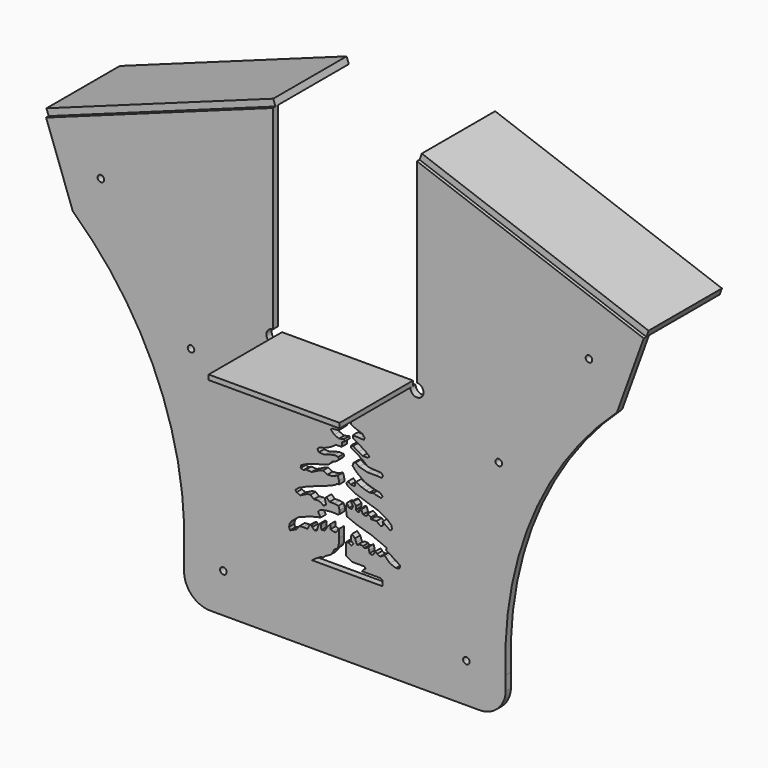
from build123d import *

# Parameters (mm, degrees)
F0_R     = 3.175
F1_DEPTH = 3.175
F2_DEPTH = 88.9
F0_W     = 127
F0_H     = 4.7752
F3_DEPTH = 88.9


# Not quite as in the source:
# - ends of sketch curves that miss each other by under 0.0002 mm in the source are joined
# - a feature names something its author has since deleted; it is built from what else it names


with BuildPart() as f1:
    # F0 (on Front) → F1 (new body, symmetric)
    with BuildSketch(Plane.XZ):
        Polygon((-69.85, 303.926875), (-203.2, 255.5875), (-69.85, 255.5875), align=None)
        Polygon((69.85, 303.926875), (69.85, 255.5875), (203.2, 255.5875), align=None)
        with BuildLine():
            Line((-167.3808159173, -1.6199540129), (-203.2, 255.5875))
            Line((-203.2, 255.5875), (-203.2, 78.7780769081))
            ThreePointArc((-203.2, 78.7780769081), (-182.9956492828, 39.6036195315), (-168.1761064252, -1.908246822))
            Line((-168.1761064252, -1.908246822), (-167.3808159173, -1.6199540129))
        make_face()
        with BuildLine():
            Line((289.7688754486, 224.2062826499), (203.2, 255.5875))
            Line((203.2, 255.5875), (203.2, 78.7780769081))
            ThreePointArc((203.2, 78.7780769081), (230.8249337186, 117.8698826041), (263.7999669887, 152.5679144845))
            Line((263.7999669887, 152.5679144845), (289.7688754486, 224.2062826499))
        make_face()
        with Locations((236.637085726, 189.4318247696)):
            Circle(F0_R, mode=Mode.SUBTRACT)
        with BuildLine():
            Line((-203.2, 78.7780769081), (-203.2, 255.5875))
            Line((-203.2, 255.5875), (-289.7688754486, 224.2062826499))
            Line((-289.7688754486, 224.2062826499), (-263.7999669887, 152.5679144845))
            ThreePointArc((-263.7999669887, 152.5679144845), (-230.8249337186, 117.8698826041), (-203.2, 78.7780769081))
        make_face()
        with Locations((-236.637085726, 189.4318247696)):
            Circle(F0_R, mode=Mode.SUBTRACT)
        with BuildLine():
            Line((203.2, 78.7780769081), (203.2, 255.5875))
            Line((203.2, 255.5875), (167.3808159173, -1.6199540129))
            Line((167.3808159173, -1.6199540129), (168.1761064252, -1.908246822))
            ThreePointArc((168.1761064252, -1.908246822), (182.9956492828, 39.6036195315), (203.2, 78.7780769081))
        make_face()
        with BuildLine():
            Line((-69.85, 255.5875), (-203.2, 255.5875))
            Line((-203.2, 255.5875), (-167.3808159173, -1.6199540129))
            Line((-167.3808159173, -1.6199540129), (-168.1761064252, -1.908246822))
            ThreePointArc((-168.1761064252, -1.908246822), (-157.8501469155, -53.8850159886), (-155.95205801, -106.8435585601))
            Line((-155.95205801, -106.8435585601), (-155.95205801, -119.5435604932))
            ThreePointArc((-155.95205801, -119.5435604932), (-148.5125702522, -137.5040727354), (-130.55205801, -144.9435604932))
            Line((-130.55205801, -144.9435604932), (130.5678750061, -144.9435585601))
            ThreePointArc((130.5678750061, -144.9435585601), (148.2086715246, -137.8181939378), (155.95205801, -120.439802512))
            Line((155.95205801, -120.439802512), (155.95205801, -118.6473146081))
            Line((155.95205801, -118.6473146081), (155.95205801, -106.8435585601))
            ThreePointArc((155.95205801, -106.8435585601), (157.8501469155, -53.8850159886), (168.1761064252, -1.908246822))
            Line((168.1761064252, -1.908246822), (167.3808159173, -1.6199540129))
            Line((167.3808159173, -1.6199540129), (203.2, 255.5875))
            Line((203.2, 255.5875), (69.85, 255.5875))
            Line((69.85, 255.5875), (69.85, 114.9223))
            ThreePointArc((69.85, 114.9223), (74.3401280605, 113.0624280605), (76.2, 108.5723))
            ThreePointArc((76.2, 108.5723), (69.85, 102.2223), (63.5, 108.5723))
            Line((63.5, 108.5723), (-63.5, 108.5723))
            ThreePointArc((-63.5, 108.5723), (-74.3401280605, 104.0821719395), (-69.85, 114.9223))
            Line((-69.85, 114.9223), (-69.85, 255.5875))
        make_face()
        with Locations((-117.85205801, -106.8435585601)):
            Circle(F0_R, mode=Mode.SUBTRACT)
        with Locations((-100.6744361574, -17.9435585601)):
            Circle(F0_R, mode=Mode.SUBTRACT)
        Polygon((36.607734859, -64.6745339036), (36.607734859, -67.2756265469), (36.607734859, -69.7801932693), (-31.9546833634, -69.7801932693), (-28.2745026052, -67.1114251018), (-24.3145544082, -64.6745339036), (-20.9638290107, -63.7607052922), (-18.8315492123, -61.9330331683), (-14.2623763531, -59.4961456954), (-12.1300965548, -57.0592544973), (-10.3024281561, -53.7085272372), (-7.2563136928, -51.5762493014), (-6.0378699563, -48.8347448409), (-5.7332566939, -42.437903583), (-5.7332566939, -34.518007189), (-8.7793711573, -38.4779572487), (-11.5208746865, -38.4779572487), (-13.9577658847, -37.564124912), (-14.2623763531, -33.2995653152), (-15.785433352, -34.8226204515), (-17.0038808137, -36.6502888501), (-18.2223245502, -38.1733439863), (-19.4407720119, -40.3056256473), (-22.7914974093, -40.9148484468), (-23.0961069465, -38.7825705111), (-23.0961069465, -35.9453856945), (-24.5961938053, -36.2300090492), (-24.619165808, -36.3456755877), (-25.837611407, -38.4779572487), (-27.0560570061, -42.7425168455), (-29.4929482043, -43.6563529074), (-31.62522614, -41.5240712464), (-32.2344489396, -39.6964028478), (-34.671343863, -40.9148484468), (-36.1943989992, -44.5701815188), (-40.1543490589, -44.2655719817), (-44.1142953932, -44.5701815188), (-46.8557998538, -48.2255220413), (-53.2526373863, -51.271636039), (-54.1664734483, -48.5301353037), (-53.5572506487, -45.4840175807), (-51.4249689877, -42.437903583), (-44.4189086556, -36.9548983872), (-32.539062202, -32.6903387904), (-23.4007202089, -30.5580608547), (-24.619165808, -29.0350038558), (-26.1422228068, -26.2935012579), (-23.7053316087, -24.1612195969), (-18.5269378126, -22.9427739978), (-13.3485421538, -22.3335511982), (-6.9517027587, -22.638162598), (-5.1240348257, -21.7243302613), (-5.1240348257, -18.3736030012), (-6.3424808905, -15.0228776038), (-10.3024281561, -14.4136548042), (-14.871600084, -14.4136548042), (-17.9891549051, -11.3546038046), (-19.4676760584, -13.0302608013), (-19.4407720119, -13.1952101365), (-18.2223245502, -18.0689916015), (-20.6592157483, -19.5920486003), (-23.4007202089, -17.7643802017), (-25.837611407, -16.8505460024), (-30.1021710038, -17.1551574022), (-33.4528945386, -14.4136548042), (-36.4990122616, -14.7182652727), (-43.2004630566, -18.0689916015), (-46.8557998538, -16.5459346026), (-48.0742454529, -15.0228776038), (-45.0281314552, -12.2813750058), (-35.8897894621, -8.0168154091), (-20.6592157483, -2.8384211473), (-9.3885958195, 1.7307501985), (-8.4747597575, 2.949195914), (-5.4286457598, 3.5584187135), (-5.7332566939, 6.6045327112), (-6.9517027587, 10.5644809082), (-8.4747597575, 9.9552581087), (-12.1300965548, 8.4322011098), (-17.0038808137, 8.1275897101), (-21.2684404105, 10.2598704398), (-25.5330000073, 8.7368125096), (-32.2344489396, 5.3860871121), (-37.7174578607, 5.6906985119), (-40.1543490589, 4.4722529128), (-42.8958497941, 5.3860871121), (-42.591240257, 7.8229783103), (-36.1943989992, 11.1737037078), (-27.6652798057, 13.6105958372), (-16.0900466144, 16.9613212347), (-12.1300965548, 20.9212694317), (-8.1701492891, 22.4443264306), (-5.7332566939, 24.8812176287), (-6.3424808905, 26.7088860273), (-10.3024281561, 27.0134974271), (-13.0439316854, 26.4042746276), (-19.745381549, 24.2719948292), (-25.2283886075, 24.5766080916), (-26.7514456064, 27.0134974271), (-24.619165808, 28.8411676884), (-19.745381549, 30.0596132874), (-13.6531544849, 32.8011140227), (-8.7793711573, 36.1518375576), (-2.9917557258, 36.45645082), (-2.9917557258, 40.4163971543), (-0.2502521093, 41.9394560158), (-0.8594739484, 43.7671244144), (-5.7332566939, 42.5486788154), (-10.3024281561, 44.3763509393), (-13.6531544849, 47.7270744741), (-12.4347088858, 48.9455200732), (-6.0378699563, 49.5547391474), (-2.6871447917, 52.6008531451), (-5.7332566939, 55.3423576057), (-9.0839844197, 57.4746392667), (-9.3885958195, 59.6069209278), (-5.7332566939, 60.5207569897), (-1.7733093118, 61.4345856011), (-0.5548630143, 63.5668635368), (-4.5148129575, 62.9576444626), (-6.9517027587, 64.1760900617), (-4.8194238916, 66.9175907969), (-1.4686983777, 70.2683180571), (2.4912513327, 74.2282643914), (2.7958622668, 79.1020467877), (4.9281413667, 80.9297189116), (7.0604202338, 80.9297189116), (8.2788737491, 77.8836086392), (6.4512053505, 69.6590989828), (5.2327592857, 64.4807070494), (5.8419806883, 58.3884753287), (10.7157630846, 56.2561973929), (16.8079920113, 54.1239194572), (19.2448850721, 51.0778054595), (18.3310490102, 49.2501333356), (14.3710998818, 49.5547428727), (7.6696490869, 49.8593561351), (7.6696490869, 47.422464937), (12.5434342772, 44.6809642017), (19.854106009, 40.1117950678), (23.8140560687, 36.7610678077), (22.2909990698, 35.2380089462), (17.4172148108, 35.2380089462), (13.1526561454, 37.3702906072), (7.9742623493, 40.721014142), (5.8419806883, 40.4164046049), (5.8419806883, 38.5887362063), (12.2388210148, 34.9333994091), (17.1126052737, 31.8872854114), (22.2909990698, 27.6227239519), (29.6016726643, 27.013503015), (35.3892855346, 26.7088916153), (36.9123443961, 24.5766099542), (35.6939025223, 22.4443301558), (29.9062859267, 22.7489434183), (21.6817781329, 22.7489434183), (13.7618780136, 24.881221354), (10.4111554101, 27.3181125522), (8.2788737491, 26.4042783529), (7.3650381528, 23.6627757549), (11.6295991465, 19.0936047584), (19.2448850721, 13.6105995625), (29.2970575392, 10.2598741651), (34.1708436608, 9.3460399657), (36.607734859, 6.9091478363), (35.0846797228, 5.0814799033), (30.5155068636, 5.9953141026), (27.4693928659, 6.9091478363), (23.8140560687, 5.9953141026), (20.4633288085, 6.9091478363), (16.5033787489, 8.1275943667), (10.7157630846, 10.8690969646), (9.801927954, 9.0414276347), (9.4973193482, 6.9091478363), (5.5373697542, 6.9091478363), (3.100479953, 9.0414276347), (1.2728092261, 7.2137597017), (3.100479953, 4.4722571038), (10.1065412164, 0.8169198991), (21.9863858074, -3.1430283561), (33.2570075989, -6.798365619), (40.8722944558, -11.0629247501), (45.1368540525, -15.0228738785), (45.7460805774, -18.3735992759), (43.9184084535, -19.592044875), (39.9584583938, -17.1551536769), (36.6305209872, -14.4322942851), (37.102624774, -17.7370272577), (35.3892855346, -18.9828220755), (32.6477847993, -17.7643764764), (30.8201164007, -15.9367080778), (25.3371130675, -16.2413194776), (25.3371130675, -14.4136510789), (21.9863858074, -12.5859826803), (21.6817781329, -14.1090396792), (20.4633288085, -15.0228738785), (17.4172148108, -14.7182624787), (15.894157812, -10.7583133504), (14.3710998818, -11.0629247501), (14.066491276, -13.8044282794), (11.934212409, -14.1090396792), (10.7157630846, -12.8905931488), (11.0203772783, -9.5398677513), (7.9742623493, -6.798365619), (5.8419806883, -7.7121998183), (7.9742623493, -10.7583133504), (6.7558162846, -13.4998159483), (4.0143127553, -13.4998159483), (1.8820336554, -9.8444800824), (1.5774228377, -11.672148481), (0.9681983502, -14.7182624787), (1.8820336554, -21.4197132736), (4.0143127553, -22.333547473), (11.6295991465, -25.3796614707), (25.946335867, -29.6442210674), (40.5676811934, -35.7364490628), (39.9584583938, -37.8687307239), (42.9591350257, -39.7909916937), (50.2884611487, -44.0955162048), (50.315245986, -44.2655682564), (53.6659732461, -46.7024594545), (52.7521446347, -49.4439639151), (49.4014173746, -50.0531904399), (43.613795191, -47.9209087789), (39.3492355943, -43.6563491821), (37.8261804581, -43.0471226573), (34.7800664604, -44.8747947812), (33.2570075989, -44.8747947812), (31.1247296631, -43.9609587193), (29.6016726643, -42.1332903206), (28.6878366023, -43.3517359197), (27.7740005404, -45.4840138555), (26.2509435415, -46.3978499174), (23.8140560687, -45.7886271179), (23.5094428062, -43.3517359197), (22.5956086069, -40.9148447216), (20.4633288085, -42.4378998578), (18.6356622726, -43.0471226573), (17.7218280733, -41.5240675211), (14.1694936901, -41.3663946092), (14.066491276, -41.5240675211), (11.934212409, -42.4378998578), (11.0203772783, -40.9148447216), (9.801927954, -37.5641174614), (6.7558162846, -34.8226167262), (6.0713343204, -36.3456718624), (6.0713343204, -40.8503381199), (8.2788737491, -42.7425131202), (6.4512053505, -44.8747947812), (3.4050908871, -43.3517359197), (1.2728092261, -43.3517359197), (1.2728092261, -55.2315823734), (7.0604272187, -58.5823096335), (18.9402718097, -58.5823096335), (20.1426781714, -60.1992271841), (18.2843375951, -61.3142289221), (16.6737716645, -63.2964596152), (16.5033787489, -63.4560883045), (34.4754569232, -63.4560883045), align=None, mode=Mode.SUBTRACT)
        with Locations((-149.2267410619, 72.5043126906)):
            Circle(F0_R, mode=Mode.SUBTRACT)
        with Locations((0, -106.8435585601)):
            Circle(F0_R, mode=Mode.SUBTRACT)
        with Locations((117.85205801, -106.8435585601)):
            Circle(F0_R, mode=Mode.SUBTRACT)
        with Locations((100.6744361574, -17.9435585601)):
            Circle(F0_R, mode=Mode.SUBTRACT)
        with Locations((149.2267410619, 72.5043126906)):
            Circle(F0_R, mode=Mode.SUBTRACT)
        with Locations((-100.6744361574, -17.9435585601)):
            Circle(F0_R)
        with Locations((100.6744361574, -17.9435585601)):
            Circle(F0_R)
        with Locations((0, -106.8435585601)):
            Circle(F0_R)
    extrude(amount=F1_DEPTH, both=True)

    # F0 (on Front) → F2 (join)
    with BuildSketch(Plane.XZ):
        Polygon((-289.7688754486, 224.2062826499), (-203.2, 255.5875), (-69.85, 303.926875), (-72.014075705, 309.8967390138), (-291.9329511536, 230.1761466637), align=None)
        Polygon((72.014075705, 309.8967390138), (69.85, 303.926875), (203.2, 255.5875), (289.7688754486, 224.2062826499), (291.9329511536, 230.1761466637), align=None)
    extrude(amount=-F2_DEPTH)

    # F0 (on Front) → F3 (join)
    with BuildSketch(Plane.XZ):
        with Locations((0, 110.9599)):
            Rectangle(F0_W, F0_H)
    extrude(amount=F3_DEPTH)


solid = f1.part
